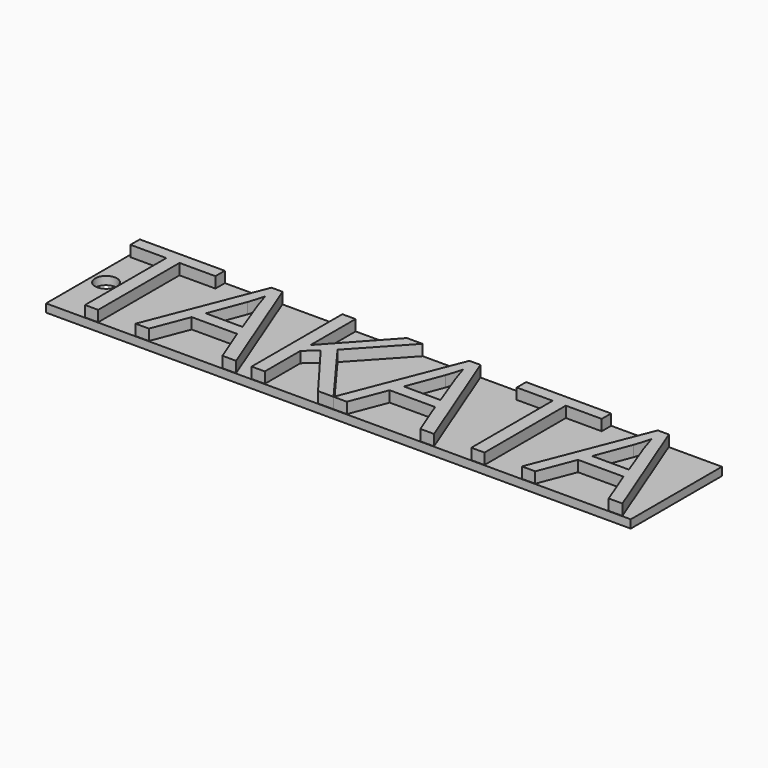
from build123d import *

# Parameters (mm, degrees)
F0_TEXT_SIZE = 73.9086108903
F2_DEPTH     = 8.89
F3_DEPTH     = 3.81
F4_D         = 10.16


# Not quite as in the source:
# - Text() gives the source's letters only with a copy of the font that has no kerning and outlines rounded to 1/6400 em; it was checked with that copy


with BuildPart() as f2:
    # F0 (on Top) → F2 (new body)
    with BuildSketch(Plane.XY):
        with Locations((-54.5351170003, -16.6058503091)):
            Text('TAKATA', F0_TEXT_SIZE, font='Open Sans', text_align=(TextAlign.LEFT, TextAlign.BOTTOM))
    extrude(amount=F2_DEPTH)


with BuildPart() as f3:
    # F1 (on Top) → F3 (new body)
    with BuildSketch(Plane.XY):
        Polygon((216.9806659222, 36.2261235714), (-55.1172271371, 36.2261235714), (-55.1172271371, 9.7051318735), (-55.1172271371, -16.8158598244), (216.9806659222, -16.8158598244), align=None)
        with BuildLine():
            ThreePointArc((-41.7273268104, 9.7051318735), (-48.4222769737, 3.0101817101), (-55.1172271371, 9.7051318735))
            ThreePointArc((-55.1172271371, 9.7051318735), (-48.4222769737, 16.4000820369), (-41.7273268104, 9.7051318735))
        make_face(mode=Mode.SUBTRACT)
        with BuildLine():
            ThreePointArc((-41.7273268104, 9.7051318735), (-48.4222769737, 16.4000820369), (-55.1172271371, 9.7051318735))
            ThreePointArc((-55.1172271371, 9.7051318735), (-48.4222769737, 3.0101817101), (-41.7273268104, 9.7051318735))
        make_face()
    extrude(amount=F3_DEPTH)

    # F4 (through all)
    with Locations(Plane(origin=(0, 0, 0), x_dir=(1, 0, 0), z_dir=(0, 0, -1))):
        with Locations((-48.4222769737, -9.7051318735)):
            Hole(F4_D / 2)


solid = Compound([f2.part, f3.part])
